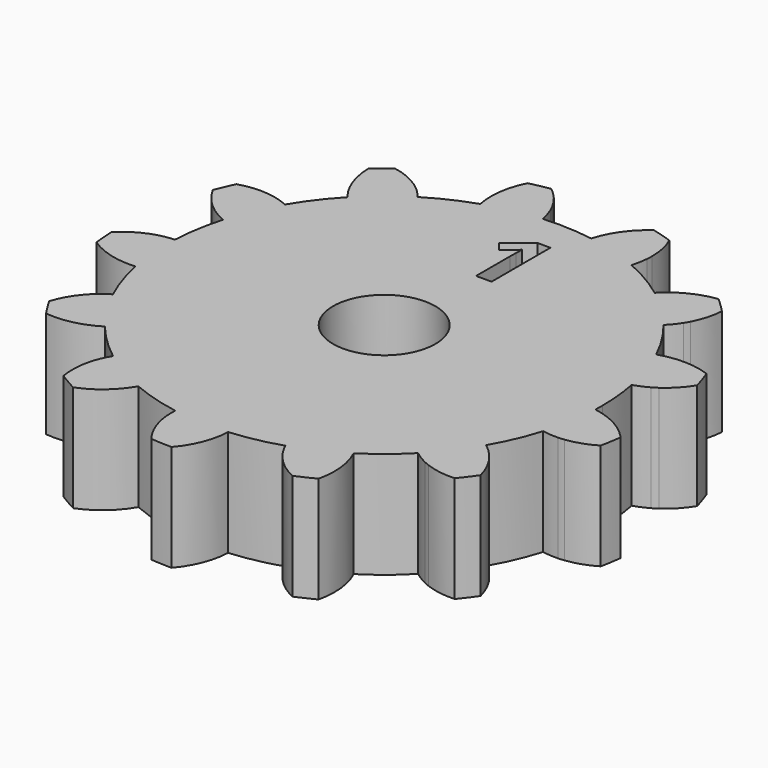
from build123d import *

# Parameters (mm, degrees)
F1_DEPTH     = 10
F2_COUNT     = 13
F3_R         = 4.8125
F4_DEPTH     = 6
F5_R         = 2
F6_DEPTH     = 4
F7_TEXT_SIZE = 9.6822995461
F8_DEPTH     = 2


# Not quite as in the source:
# - Text() gives the source's letters only with a copy of the font that has no kerning and outlines rounded to 1/6400 em; it was checked with that copy


with BuildPart() as f1:
    # F0 (on Top) → F1 (new body)
    with BuildSketch(Plane.XY):
        with BuildLine():
            ThreePointArc((7.9284276206, 23.5955864404), (6.9900144894, 23.8904031242), (6.04068631, 24.1479144628))
            ThreePointArc((6.04068631, 24.1479144628), (4.3213940573, 22.4329291679), (3.263536476, 20.2470477097))
            ThreePointArc((3.263536476, 20.2470477097), (5.7825841651, 19.676263153), (8.2099093234, 18.7933764979))
            ThreePointArc((8.2099093234, 18.7933764979), (8.3945552331, 19.5156155745), (8.498494095, 20.2538026162))
            ThreePointArc((8.498494095, 20.2538026162), (8.5166436171, 20.5392033965), (8.5226970743, 20.825116611))
            ThreePointArc((8.5226970743, 20.825116611), (8.3724590035, 22.2418610533), (7.9284276206, 23.5955864404))
        make_face()
        with BuildLine():
            ThreePointArc((4.0253666655, 14.4585201562), (-1.7454613083, 15.0554452906), (-4.9249243377, 19.9082578735))
            ThreePointArc((-4.9249243377, 19.9082578735), (-12.6410323189, -16.1492387809), (20.5083790508, 0))
            ThreePointArc((20.5083790508, 0), (19.2412101906, 7.0971432063), (15.5962949152, 13.3172518264))
            ThreePointArc((15.5962949152, 13.3172518264), (9.5252611173, 10.9925929993), (4.0253666655, 14.4585201562))
        make_face()
        with BuildLine():
            ThreePointArc((3.263536476, 20.2470477097), (-0.8477895051, 20.4908483047), (-4.9249243377, 19.9082578735))
            ThreePointArc((-4.9249243377, 19.9082578735), (-1.7454613083, 15.0554452906), (4.0253666655, 14.4585201562))
            ThreePointArc((4.0253666655, 14.4585201562), (3.0372062455, 17.2728641577), (3.263536476, 20.2470477097))
        make_face()
        with BuildLine():
            ThreePointArc((4.0253666655, 14.4585201562), (9.5252611173, 10.9925929993), (15.5962949152, 13.3172518264))
            ThreePointArc((15.5962949152, 13.3172518264), (12.2139602675, 16.4746103406), (8.2099093234, 18.7933764979))
            ThreePointArc((8.2099093234, 18.7933764979), (6.6277035692, 16.133569575), (4.0253666655, 14.4585201562))
        make_face()
        with BuildLine():
            ThreePointArc((8.2099093234, 18.7933764979), (5.7825841651, 19.676263153), (3.263536476, 20.2470477097))
            ThreePointArc((3.263536476, 20.2470477097), (3.0372062455, 17.2728641577), (4.0253666655, 14.4585201562))
            ThreePointArc((4.0253666655, 14.4585201562), (6.6277035692, 16.133569575), (8.2099093234, 18.7933764979))
        make_face()
    extrude(amount=F1_DEPTH)

    # F2: F1 ×13 about axis
    f2_axis = Axis((0, 0, 10), (0, 0, 1))


with BuildPart() as f1_1:
    add(f1.part)
    for i in range(1, F2_COUNT):
        add(f1.part.rotate(f2_axis, i * 360 / F2_COUNT))

    # F3 (on face) → F4 (cut)
    with BuildSketch(Plane.XY.offset(10)):
        Circle(F3_R)
    extrude(amount=-F4_DEPTH, mode=Mode.SUBTRACT)

    # F5 (on face) → F6 (join)
    with BuildSketch(Plane(origin=(0, 0, 0), x_dir=(1, 0, 0), z_dir=(0, 0, -1))):
        Circle(F5_R)
    extrude(amount=F6_DEPTH)

    # F7 (on face) → F8 (cut)
    with BuildSketch(Plane.XY.offset(10)):
        with Locations((-2.153794514, 10.3121809661)):
            Text('1', F7_TEXT_SIZE, font='Open Sans', font_style=FontStyle.BOLD, text_align=(TextAlign.LEFT, TextAlign.BOTTOM))
    extrude(amount=-F8_DEPTH, mode=Mode.SUBTRACT)


solid = f1_1.part
